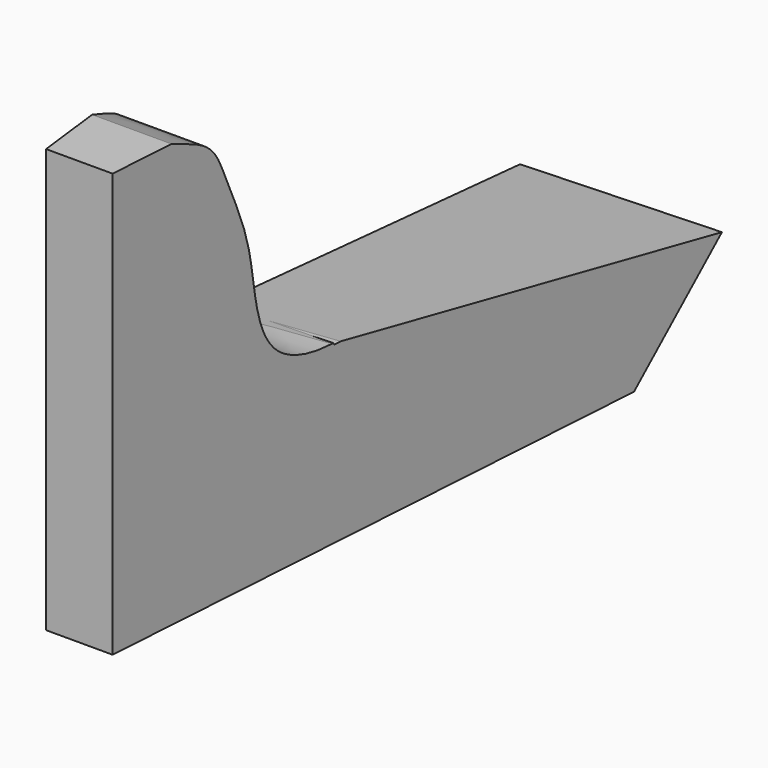
from build123d import *

# Parameters (mm, degrees)
F0_W      = 25.1408442855
F0_H      = 121.0211291909
F1_DEPTH  = 50
F2_SIZE   = 49.99999
F3_W      = 91.4516113698
F3_H      = 29.3820567429
F4_DEPTH  = 26
F7_DEPTH  = 26
F9_DEPTH  = 50
F11_DEPTH = 55
F13_DEPTH = 25


# Not quite as in the source:
# - a fillet or chamfer is up to 0.001 mm smaller than in the source, because OpenCascade refuses the exact size


with BuildPart() as f1:
    # F0 (on Top) → F1 (new body)
    with BuildSketch(Plane.XY):
        with Locations((-35.985916853, -13.0633823574)):
            Rectangle(F0_W, F0_H)
    extrude(amount=F1_DEPTH)

    # F2 (size 50 in the source; OpenCascade refuses exactly that, so slightly less here)
    f2_edges = [f1.edges().sort_by_distance(p)[0] for p in [
        (-35.985917, 47.447182, 0),
    ]]
    chamfer(f2_edges, length=F2_SIZE)

    # F3 (on face) → F4 (cut)
    with BuildSketch(Plane.YZ.offset(-23.4154947102)):
        with Locations((2.2862907499, 35.3089716285)):
            Rectangle(F3_W, F3_H)
    extrude(amount=-F4_DEPTH, mode=Mode.SUBTRACT)

    # F6 (on face) → F7 (cut)
    with BuildSketch(Plane.YZ.offset(-23.4154947102)):
        with BuildLine():
            add(Edge.make_bspline(
                [(-66.471672154, 50.7267448454), (-66.3301689203, 49.9168473843), (-59.8711260209, 48.6776696356), (-58.2068726445, 43.1050844178), (-54.0340520057, 35.0412473829), (-54.2777638398, 19.262544423), (-29.8031687904, 20.774326267), (-23.5577770812, 45.5234958201), (-47.8291550907, 56.2410515184), (-66.7088060402, 52.0839868491), (-66.471672154, 50.7267448454)],
                knots=[0, 0, 0, 0, 0.0838937014, 0.1662578753, 0.2711363939, 0.393677104, 0.5393220763, 0.6884110648, 0.8594092945, 1, 1, 1, 1], degree=3))
        make_face()
    extrude(amount=-F7_DEPTH, mode=Mode.SUBTRACT)

    # F8 (on Top) → F9 (cut)
    with BuildSketch(Plane.XY):
        Polygon((-37.4647900462, -76.7781734467), (-49.2957793176, 19.8415517807), (-59.1298444312, -76.7781734467), align=None)
    extrude(amount=F9_DEPTH, mode=Mode.SUBTRACT)

    # F10 (on Top) → F11 (cut)
    with BuildSketch(Plane.XY):
        Polygon((-11.8309855461, -74.559867382), (-23.4154947102, 25.2640862018), (-30.0704240799, -74.559867382), align=None)
    extrude(amount=F11_DEPTH, mode=Mode.SUBTRACT)

    # F12 (on face) → F13 (cut)
    with BuildSketch(Plane(origin=(-46.1738809914, -5.6539458102, 0), x_dir=(0.1215412158, -0.9925863856, 0), z_dir=(-0.9925863856, -0.1215412158, 0))):
        Polygon((-24.7206917847, 26.6503777788), (-24.7206917847, 9.8842468545), (40.7590243896, 20.9504020134), align=None)
    extrude(amount=-F13_DEPTH, mode=Mode.SUBTRACT)


solid = f1.part
